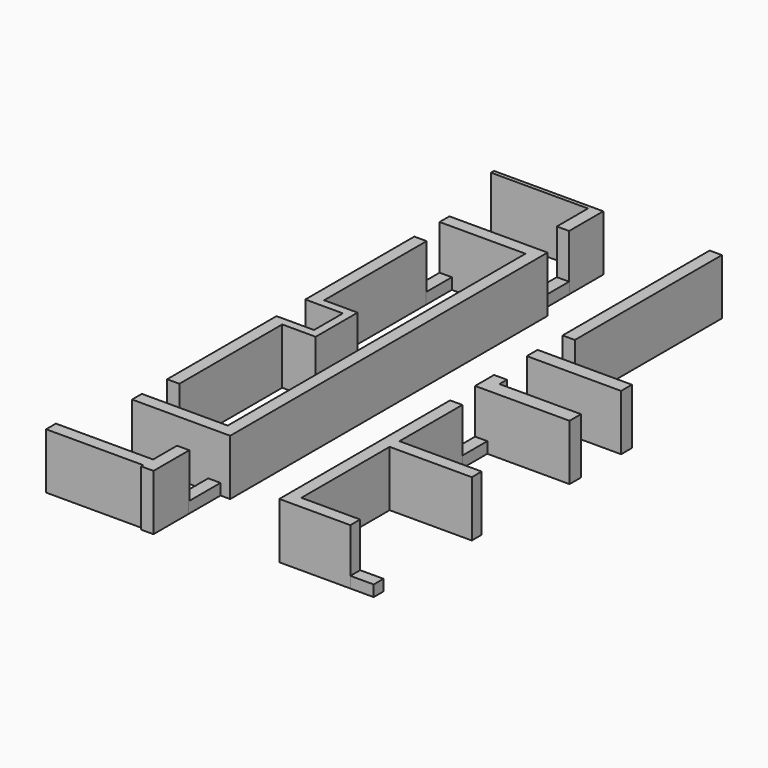
from build123d import *

# Parameters (mm, degrees)
F1_DEPTH = 3.81
F0_W     = 0.0016617535
F0_H     = 0.8382
F0_W_2   = 5.6088228764
F0_W_3   = 0.0049910592
F0_H_2   = 0.9810682386
F0_W_4   = 5.5669181896
F0_W_5   = 0.8382
F0_H_3   = 12.5598123049
F0_W_6   = 6.4442373921
F0_H_4   = 0.9225998074
F0_W_7   = 5.8674
F0_W_8   = 0.5588
F0_H_5   = 2.4610901317
F0_W_9   = 6.6410191357
F2_W     = 0.8382
F2_H     = 2.2369018
F3_DEPTH = 0.762
F2_H_2   = 2.8956
F2_H_3   = 2.2606
F2_W_2   = 1.6959072
F2_H_4   = 0.8382
F2_H_5   = 2.7686


# Not quite as in the source:
# - ends of sketch curves that miss each other by under 0.0002 mm in the source are joined


with BuildPart() as f1:
    # F0 (on Top) → F1 (new body)
    with BuildSketch(Plane.XY):
        Polygon((-47.496972236, -2.1997114257), (-47.496972236, 0.7173087654), (-48.335172236, 0.7173087654), (-48.335172236, 0.4585053894), (-48.335172236, -2.1997114257), align=None)
        Polygon((-48.335172236, 0.4585053894), (-48.335172236, 0.7173087654), (-54.9666435823, 0.7173984171), (-54.9666435823, 0.4585053894), align=None)
    extrude(amount=F1_DEPTH)


with BuildPart() as f1b:
    # F0 (on Top) → F1, piece 2 (new body)
    with BuildSketch(Plane.XY):
        with Locations((-33.7847184829, -27.2344640045)):
            Rectangle(F0_W, F0_H)
        with Locations((-36.5899607978, -27.2344640045)):
            Rectangle(F0_W_2, F0_H)
        Polygon((-39.394372236, -27.6535640045), (-39.394372236, -26.8153640045), (-39.394372236, -21.4452373369), (-40.232572236, -21.4452373369), (-40.232572236, -35.1905039115), (-39.394372236, -35.1905039115), align=None)
        Polygon((-35.379845649, -35.1905039115), (-39.394372236, -35.1905039115), (-40.232572236, -35.1905039115), (-40.232572236, -36.0287039115), (-35.379845649, -36.0287039115), align=None)
    extrude(amount=F1_DEPTH)


with BuildPart() as f1c:
    # F0 (on Top) → F1, piece 3 (new body)
    with BuildSketch(Plane.XY):
        with Locations((-33.78305383, -18.8194096594)):
            Rectangle(F0_W_3, F0_H_2)
        with Locations((-36.5690084544, -18.8194096594)):
            Rectangle(F0_W_4, F0_H_2)
        Polygon((-39.3524675492, -19.3099437787), (-39.3524675492, -18.3288755401), (-39.3524675492, -17.690040408), (-40.232572236, -17.690040408), (-40.232572236, -19.3099437787), align=None)
    extrude(amount=F1_DEPTH)


with BuildPart() as f1d:
    # F0 (on Top) → F1, piece 4 (new body)
    with BuildSketch(Plane.XY):
        with Locations((-39.813472236, -5.5599344481)):
            Rectangle(F0_W_5, F0_H_3)
    extrude(amount=F1_DEPTH)


with BuildPart() as f1e:
    # F0 (on Top) → F1, piece 5 (new body)
    with BuildSketch(Plane.XY):
        with Locations((-37.0104535399, -14.4347405043)):
            Rectangle(F0_W_6, F0_H_4)
    extrude(amount=F1_DEPTH)


with BuildPart() as f1f:
    # F0 (on Top) → F1, piece 6 (new body)
    with BuildSketch(Plane.XY):
        Polygon((-46.836572236, -4.8667114257), (-53.542172236, -4.8667114257), (-53.542172236, -5.7049114257), (-47.674772236, -5.7049114257), (-46.836572236, -5.7049114257), align=None)
        Polygon((-46.836572236, -31.9681875408), (-46.836572236, -5.7049114257), (-47.674772236, -5.7049114257), (-47.674772236, -31.1299875408), (-47.674772236, -31.9681875408), align=None)
        with Locations((-50.608472236, -31.5490875408)):
            Rectangle(F0_W_7, F0_H)
    extrude(amount=F1_DEPTH)


with BuildPart() as f1g:
    # F0 (on Top) → F1, piece 7 (new body)
    with BuildSketch(Plane.XY):
        Polygon((-52.703972236, -7.8639114257), (-53.542172236, -7.8639114257), (-53.542172236, -17.1703245472), (-52.703972236, -17.1703245472), (-52.703972236, -16.6115245472), align=None)
        Polygon((-50.417972236, -16.6115245472), (-52.703972236, -16.6115245472), (-52.703972236, -17.1703245472), (-50.976772236, -17.1703245472), (-50.417972236, -17.1703245472), align=None)
        with Locations((-50.697372236, -18.4008696131)):
            Rectangle(F0_W_8, F0_H_5)
        Polygon((-50.417972236, -19.631414679), (-50.976772236, -19.631414679), (-52.703972236, -19.631414679), (-52.703972236, -20.190214679), (-50.417972236, -20.190214679), align=None)
        Polygon((-52.703972236, -20.190214679), (-52.703972236, -19.631414679), (-53.542172236, -19.631414679), (-53.542172236, -28.9709875408), (-52.703972236, -28.9709875408), align=None)
    extrude(amount=F1_DEPTH)


with BuildPart() as f1h:
    # F0 (on Top) → F1, piece 8 (new body)
    with BuildSketch(Plane.XY):
        Polygon((-47.496972236, -34.6351875408), (-48.335172236, -34.6351875408), (-48.335172236, -36.6773806541), (-48.335172236, -37.5155806541), (-48.335172236, -37.6932546496), (-47.496972236, -37.6932546496), align=None)
        with Locations((-51.6556818038, -37.0964806541)):
            Rectangle(F0_W_9, F0_H)
    extrude(amount=F1_DEPTH)


with BuildPart() as f3:
    # F2 (on Top) → F3 (new body)
    with BuildSketch(Plane.XY):
        with Locations((-39.8135535358, -12.9074915006)):
            Rectangle(F2_W, F2_H)
    extrude(amount=F3_DEPTH)


with BuildPart() as f3b:
    # F2 (on Top) → F3, piece 2 (new body)
    with BuildSketch(Plane.XY):
        with Locations((-39.813451476, -16.293040408)):
            Rectangle(F2_W, F2_H_2)
    extrude(amount=F3_DEPTH)


with BuildPart() as f3c:
    # F2 (on Top) → F3, piece 3 (new body)
    with BuildSketch(Plane.XY):
        with Locations((-53.1226970702, -6.7844114257)):
            Rectangle(F2_W, F2_H_3)
    extrude(amount=F3_DEPTH)


with BuildPart() as f3d:
    # F2 (on Top) → F3, piece 4 (new body)
    with BuildSketch(Plane.XY):
        with Locations((-53.1230546267, -30.0504875408)):
            Rectangle(F2_W, F2_H_3)
    extrude(amount=F3_DEPTH)


with BuildPart() as f3e:
    # F2 (on Top) → F3, piece 5 (new body)
    with BuildSketch(Plane.XY):
        with Locations((-34.633492049, -35.6095951541)):
            Rectangle(F2_W_2, F2_H_4)
    extrude(amount=F3_DEPTH)


with BuildPart() as f3f:
    # F2 (on Top) → F3, piece 6 (new body)
    with BuildSketch(Plane.XY):
        with Locations((-39.8135408784, -20.3775946787)):
            Rectangle(F2_W, F2_H)
    extrude(amount=F3_DEPTH)


with BuildPart() as f3g:
    # F2 (on Top) → F3, piece 7 (new body)
    with BuildSketch(Plane.XY):
        with Locations((-47.9158710703, -3.5332114257)):
            Rectangle(F2_W, F2_H_5)
    extrude(amount=F3_DEPTH)


with BuildPart() as f3h:
    # F2 (on Top) → F3, piece 8 (new body)
    with BuildSketch(Plane.XY):
        with Locations((-47.9160200819, -33.3016875408)):
            Rectangle(F2_W, F2_H_5)
    extrude(amount=F3_DEPTH)


solid = Compound([f1.part, f1b.part, f1c.part, f1d.part, f1e.part, f1f.part, f1g.part, f1h.part, f3.part, f3b.part, f3c.part, f3d.part, f3e.part, f3f.part, f3g.part, f3h.part])
